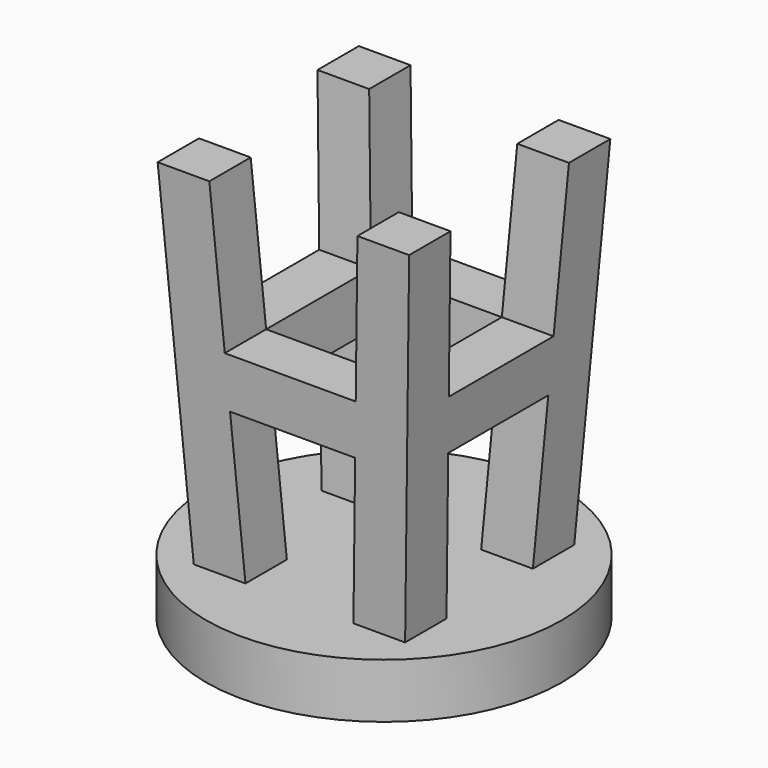
from build123d import *

# Parameters (mm, degrees)
F0_R     = 8.255
F1_DEPTH = 2.54
F8_DEPTH = 33.656
F9_W     = 6.078346395
F9_H     = 6.078346395
F10_W    = 5.8075642901
F10_H    = 5.8075642901


# Not quite as in the source:
# - a pattern or mirror of a feature is missing from the dataset's text; its kind, count and spacing are read off the source's solid


with BuildPart() as f1:
    # F0 (on Top) → F1 (new body)
    with BuildSketch(Plane.XY):
        Circle(F0_R)
    extrude(amount=F1_DEPTH)

    # F2 (on Top) → F5 section 0
    with BuildSketch(Plane.XY):
        Polygon((4.7625, 2.3625), (4.7625, 4.7625), (2.3625, 4.7625), (-2.3625, 4.7625), (-4.7625, 4.7625), (-4.7625, 2.3625), (-4.7625, -2.3625), (-4.7625, -4.7625), (-2.3625, -4.7625), (2.3625, -4.7625), (4.7625, -4.7625), (4.7625, -2.3625), align=None)
    # F4 (on offset) → F5 section 1
    with BuildSketch(Plane.XY.offset(19.05)):
        Polygon((-3.4371664787, 5.8371664787), (-5.8371664787, 5.8371664787), (-5.8371664787, 3.4371664787), (-5.8371664787, -3.4371664787), (-5.8371664787, -5.8371664787), (-3.4371664787, -5.8371664787), (3.4371664787, -5.8371664787), (5.8371664787, -5.8371664787), (5.8371664787, -3.4371664787), (5.8371664787, 3.4371664787), (5.8371664787, 5.8371664787), (3.4371664787, 5.8371664787), align=None)
    loft()

    # F7 (on offset) → F8 (cut, through all)
    with BuildSketch(Plane.XZ.offset(25.4)):
        Polygon((3.0391731975, 11.995), (3.4371664787, 19.05), (-3.4371664787, 19.05), (-3.0391731975, 11.995), align=None)
        Polygon((-2.5057888638, 2.54), (2.5057888638, 2.54), (2.903782145, 9.595), (-2.903782145, 9.595), align=None)
    f8 = extrude(amount=-F8_DEPTH, mode=Mode.SUBTRACT)

    # F8_copies: F8 across plane
    add(f8.mirror(Plane(origin=(0, 0, 0), x_dir=(0.7071067812, -0.7071067812, 0), z_dir=(0.7071067812, 0.7071067812, 0))), mode=Mode.SUBTRACT)

    # F9 (on face) → F11 section 0
    with BuildSketch(Plane.XY.offset(11.995)):
        Rectangle(F9_W, F9_H)
    # F10 (on face) → F11 section 1
    with BuildSketch(Plane(origin=(0, 0, 9.595), x_dir=(1, 0, 0), z_dir=(0, 0, -1))):
        Rectangle(F10_W, F10_H)
    loft(mode=Mode.SUBTRACT)


solid = f1.part
